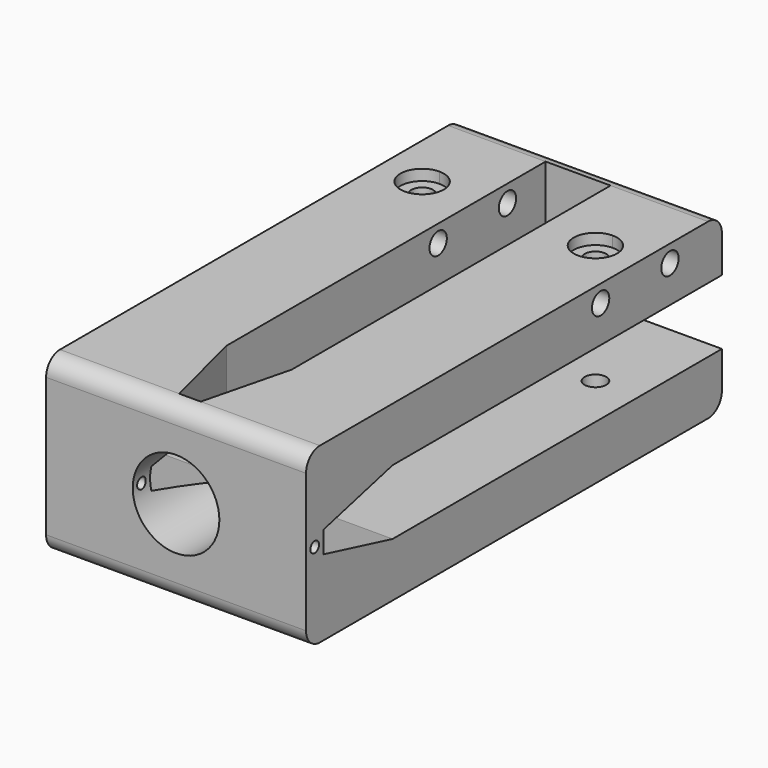
from build123d import *

# Parameters (mm, degrees)
F0_W      = 76.2
F0_H      = 50.8
F0_R      = 12.7
F1_DEPTH  = 152.4
F2_R      = 5.08
F4_DEPTH  = 76.201
F5_W      = 19.05
F5_H      = 116.84
F6_DEPTH  = 19.05
F8_DEPTH  = 50.801
F10_DEPTH = 76.201
F12_DEPTH = 3.175
F13_R     = 3.175
F14_DEPTH = 47.6260001
F15_R     = 3.175
F16_DEPTH = 47.6260001
F17_R     = 6.35
F18_DEPTH = 6.35
F19_R     = 3.175
F20_DEPTH = 76.2010001


with BuildPart() as f1:
    # F0 (on Front) → F1 (new body)
    with BuildSketch(Plane.XZ):
        Rectangle(F0_W, F0_H)
        Circle(F0_R, mode=Mode.SUBTRACT)
    extrude(amount=F1_DEPTH)

    # F2
    f2_edges = [f1.edges().sort_by_distance(p)[0] for p in [
        (0, -152.4, 25.4),
        (0, -152.4, -25.4),
        (0, 0, 25.4),
        (0, 0, -25.4),
    ]]
    fillet(f2_edges, radius=F2_R)

    # F3 (on face) → F4 (cut, through all)
    with BuildSketch(Plane(origin=(-38.1, 0, 0), x_dir=(0, -1, 0), z_dir=(-1, 0, 0))):
        Polygon((12.7, 0), (0, 0), (0, -3.175), (0, -9.525), (120.65, -9.525), (120.65, 0), (88.9, 0), align=None)
        Polygon((0, 3.175), (0, 0), (12.7, 0), (88.9, 0), (120.65, 0), (120.65, 9.525), (0, 9.525), align=None)
        Polygon((120.65, 9.525), (120.65, 0), (139.7, 0), (146.05, 0), (146.05, 3.175), align=None)
        Polygon((139.7, 0), (120.65, 0), (120.65, -9.525), (146.05, -3.175), (146.05, 0), align=None)
    extrude(amount=-F4_DEPTH, mode=Mode.SUBTRACT)

    # F5 (on face) → F6 (cut)
    with BuildSketch(Plane.XY.offset(25.4)):
        Polygon((-3.175, -147.32), (0, -147.32), (3.175, -147.32), (9.525, -121.92), (-9.525, -121.92), align=None)
        with Locations((0, -63.5)):
            Rectangle(F5_W, F5_H)
    extrude(amount=-F6_DEPTH, mode=Mode.SUBTRACT)

    # F7 (on face) → F8 (cut, through all)
    with BuildSketch(Plane(origin=(0, 0, -25.4), x_dir=(1, 0, 0), z_dir=(0, 0, -1))):
        with BuildLine():
            ThreePointArc((0, 20.955), (-3.175, 17.78), (0, 14.605))
            Line((0, 14.605), (0, 17.78))
            Line((0, 17.78), (0, 20.955))
        make_face()
        with BuildLine():
            ThreePointArc((0, 71.755), (-3.175, 68.58), (0, 65.405))
            Line((0, 65.405), (0, 68.58))
            Line((0, 68.58), (0, 71.755))
        make_face()
        with BuildLine():
            Line((0, 68.58), (0, 65.405))
            ThreePointArc((0, 65.405), (2.2450640303, 66.3349359697), (3.175, 68.58))
            ThreePointArc((3.175, 68.58), (2.2450640303, 70.8250640303), (0, 71.755))
            Line((0, 71.755), (0, 68.58))
        make_face()
        with BuildLine():
            Line((0, 17.78), (0, 14.605))
            ThreePointArc((0, 14.605), (2.2450640303, 15.5349359697), (3.175, 17.78))
            ThreePointArc((3.175, 17.78), (2.2450640303, 20.0250640303), (0, 20.955))
            Line((0, 20.955), (0, 17.78))
        make_face()
    extrude(amount=-F8_DEPTH, mode=Mode.SUBTRACT)

    # F9 (on face) → F10 (cut, through all)
    with BuildSketch(Plane(origin=(-38.1, 0, 0), x_dir=(0, -1, 0), z_dir=(-1, 0, 0))):
        with BuildLine():
            ThreePointArc((147.6375, 0), (149.225, -1.5875), (150.8125, 0))
            Line((150.8125, 0), (149.225, 0))
            Line((149.225, 0), (147.6375, 0))
        make_face()
        with BuildLine():
            Line((149.225, 0), (150.8125, 0))
            ThreePointArc((150.8125, 0), (149.225, 1.5875), (147.6375, 0))
            Line((147.6375, 0), (149.225, 0))
        make_face()
    extrude(amount=-F10_DEPTH, mode=Mode.SUBTRACT)

    # F11 (on face) → F12 (cut)
    with BuildSketch(Plane.XY.offset(25.4)):
        with BuildLine():
            ThreePointArc((-19.05, -30.48), (-20.9098719395, -25.9898719395), (-25.4, -24.13))
            ThreePointArc((-25.4, -24.13), (-29.8901280605, -34.9701280605), (-19.05, -30.48))
        make_face()
        with BuildLine():
            ThreePointArc((31.75, -30.48), (29.8901280605, -25.9898719395), (25.4, -24.13))
            ThreePointArc((25.4, -24.13), (20.9098719395, -34.9701280605), (31.75, -30.48))
        make_face()
    extrude(amount=-F12_DEPTH, mode=Mode.SUBTRACT)

    # F13 (on face) → F14 (cut, through all)
    with BuildSketch(Plane.XY.offset(22.225)):
        with Locations((25.4, -30.48)):
            Circle(F13_R)
    extrude(amount=-F14_DEPTH, mode=Mode.SUBTRACT)

    # F15 (on face) → F16 (cut, through all)
    with BuildSketch(Plane.XY.offset(22.225)):
        with Locations((-25.4, -30.48)):
            Circle(F15_R)
    extrude(amount=-F16_DEPTH, mode=Mode.SUBTRACT)

    # F17 (on face) → F18 (cut)
    with BuildSketch(Plane(origin=(0, 0, -25.4), x_dir=(1, 0, 0), z_dir=(0, 0, -1))):
        with Locations((-25.4, 30.48)):
            Circle(F17_R)
        with Locations((25.4, 30.48)):
            Circle(F17_R)
    extrude(amount=-F18_DEPTH, mode=Mode.SUBTRACT)

    # F19 (on face) → F20 (cut, through all)
    with BuildSketch(Plane(origin=(-38.1, 0, 0), x_dir=(0, -1, 0), z_dir=(-1, 0, 0))):
        with BuildLine():
            ThreePointArc((47.625, 20.32), (44.45, 23.495), (41.275, 20.32))
            ThreePointArc((41.275, 20.32), (44.45, 17.145), (47.625, 20.32))
        make_face()
        with Locations((19.05, 20.32)):
            Circle(F19_R)
    extrude(amount=-F20_DEPTH, mode=Mode.SUBTRACT)


solid = f1.part
